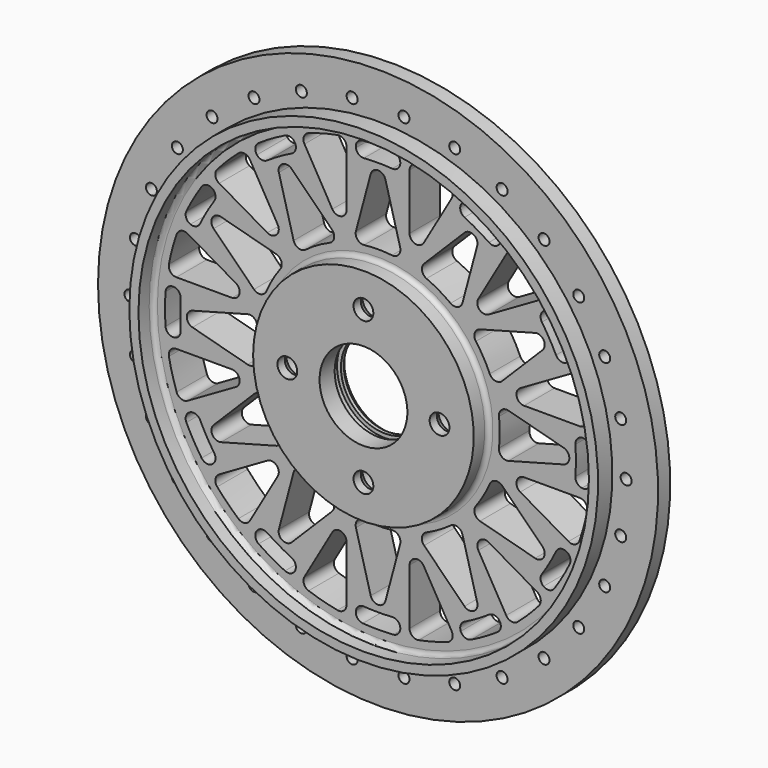
from build123d import *

# Parameters (mm, degrees)
F2_R            = 3.6
F3_DEPTH        = 50
F3_COPIES_COUNT = 30
F5_COPIES_COUNT = 4
F7_DEPTH        = 37.001
F7_COPIES_COUNT = 12


# Not quite as in the source:
# - a pattern or mirror of a feature is missing from the dataset's text; its kind, count and spacing are read off the source's solid


with BuildPart() as f1:
    # F0 (on Top) → F1 (revolve)
    with BuildSketch(Plane.XY):
        with BuildLine():
            ThreePointArc((-75.5, 12), (-73.3786796564, 11.1213203436), (-72.5, 9))
            Line((-72.5, 9), (-72.5, 0))
            Line((-72.5, 0), (-28.85, 0))
            Line((-28.85, 0), (-28.85, 12.4))
            Line((-28.85, 12.4), (-31.45, 12.4))
            Line((-31.45, 12.4), (-31.45, 17.6))
            Line((-31.45, 17.6), (-28.85, 17.6))
            Line((-28.85, 17.6), (-28.85, 20))
            Line((-28.85, 20), (-30, 20))
            ThreePointArc((-30, 20), (-30.7071067812, 20.2928932188), (-31, 21))
            Line((-31, 21), (-31, 23))
            Line((-31, 23), (-67.5, 37))
            Line((-67.5, 37), (-154, 37))
            Line((-154, 37), (-154, 22))
            Line((-154, 22), (-184, 22))
            Line((-184, 22), (-184, 12))
            Line((-184, 12), (-154, 12))
            Line((-154, 12), (-154, 0.2))
            Line((-154, 0.2), (-148, 0.2))
            Line((-148, 0.2), (-148, 9))
            ThreePointArc((-148, 9), (-147.1213203436, 11.1213203436), (-145, 12))
            Line((-145, 12), (-75.5, 12))
        make_face()
    revolve(axis=Axis((0, 8.013517431, 0), (0, -1, 0)))

    # F2 (on Front) → F3 (cut)
    with BuildSketch(Plane.XZ):
        with Locations((163, 0)):
            Circle(F2_R)
    f3 = extrude(amount=-F3_DEPTH, mode=Mode.SUBTRACT)

    # F3_copies: F3 ×30 about axis
    f3_copies_axis = Axis((0, 0, 0), (0, 1, 0))
    for i in range(1, F3_COPIES_COUNT):
        add(f3.rotate(f3_copies_axis, i * 360 / F3_COPIES_COUNT), mode=Mode.SUBTRACT)

    # F4 (on Right) → F5 (revolve, cut)
    with BuildSketch(Plane.YZ):
        Polygon((0, 56.5), (0, 50), (51.0571013514, 50), (51.0571013514, 59), (10.3301270189, 59), (6, 56.5), align=None)
    f5 = revolve(axis=Axis((0, 25.5285506757, 50), (0, 1, 0)), mode=Mode.SUBTRACT)

    # F5_copies: F5 ×4 about axis
    f5_copies_axis = Axis((0, 0, 0), (0, 1, 0))
    for i in range(1, F5_COPIES_COUNT):
        add(f5.rotate(f5_copies_axis, i * 360 / F5_COPIES_COUNT), mode=Mode.SUBTRACT)

    # F6 (on face) → F7 (cut, through all)
    with BuildSketch(Plane(origin=(0, 37, 0), x_dir=(-1, 0, 0), z_dir=(0, 1, 0))):
        with BuildLine():
            ThreePointArc((-9.1387464491, 79.4763066161), (0, 80), (9.1387464491, 79.4763066161))
            ThreePointArc((9.1387464491, 79.4763066161), (13.4960488483, 81.1778118608), (14.5395472336, 85.7376710051))
            Line((14.5395472336, 85.7376710051), (4.8296291314, 121.9755786997))
            ThreePointArc((4.8296291314, 121.9755786997), (0, 125.6814834742), (-4.8296291314, 121.9755786997))
            Line((-4.8296291314, 121.9755786997), (-14.5395472336, 85.7376710051))
            ThreePointArc((-14.5395472336, 85.7376710051), (-13.4960488483, 81.1778118608), (-9.1387464491, 79.4763066161))
        make_face()
        with BuildLine():
            ThreePointArc((-20.7055236082, 132.5300949069), (-22.5243510374, 136.3875734972), (-26.6575800381, 137.4386169405))
            ThreePointArc((-26.6575800381, 137.4386169405), (-36.2346663144, 135.2296156805), (-45.6331669538, 132.3541237505))
            ThreePointArc((-45.6331669538, 132.3541237505), (-48.6871265465, 129.3772789278), (-48.3335380101, 125.1271907594))
            Line((-48.3335380101, 125.1271907594), (-30.0356506271, 93.434320141))
            ThreePointArc((-30.0356506271, 93.434320141), (-24.4114283827, 91.1046910095), (-20.7055236082, 95.934320141))
            Line((-20.7055236082, 95.934320141), (-20.7055236082, 132.5300949069))
        make_face()
        with BuildLine():
            ThreePointArc((-9.2857142857, 129.6679432636), (0, 130), (9.2857142857, 129.6679432636))
            ThreePointArc((9.2857142857, 129.6679432636), (12.7862012081, 130.7668061158), (14.5941974866, 133.9593063458))
            ThreePointArc((14.5941974866, 133.9593063458), (13.5312228777, 137.7985159158), (10, 139.6424004377))
            ThreePointArc((10, 139.6424004377), (0, 140), (-10, 139.6424004377))
            ThreePointArc((-10, 139.6424004377), (-13.5312228777, 137.7985159158), (-14.5941974866, 133.9593063458))
            ThreePointArc((-14.5941974866, 133.9593063458), (-12.7862012081, 130.7668061158), (-9.2857142857, 129.6679432636))
        make_face()
    f7 = extrude(amount=-F7_DEPTH, mode=Mode.SUBTRACT)

    # F7_copies: F7 ×12 about axis
    f7_copies_axis = Axis((0, 0, 0), (0, 1, 0))
    for i in range(1, F7_COPIES_COUNT):
        add(f7.rotate(f7_copies_axis, i * 360 / F7_COPIES_COUNT), mode=Mode.SUBTRACT)


solid = f1.part
